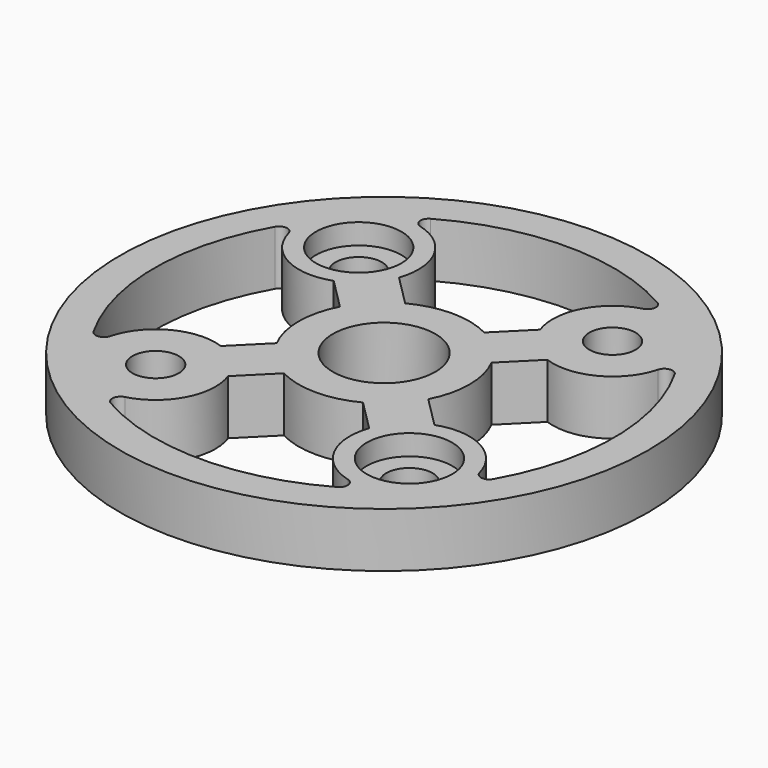
from build123d import *

# Parameters (mm, degrees)
F0_R            = 24.51608
F0_R_2          = 2.15265
F0_R_3          = 4.7625
F1_DEPTH        = 5.08
F3_DEPTH        = 5.08
F3_COPIES_COUNT = 4
F4_R            = 0.762
F6_R            = 3.96875
F7_DEPTH        = 1.905


# Not quite as in the source:
# - a pattern or mirror of a feature is missing from the dataset's text; its kind, count and spacing are read off the source's solid


with BuildPart() as f1:
    # F0 (on Top) → F1 (new body)
    with BuildSketch(Plane.XY):
        Circle(F0_R)
        with Locations((-11.7865906, -11.7865906)):
            Circle(F0_R_2, mode=Mode.SUBTRACT)
        with Locations((11.7865906, -11.7865906)):
            Circle(F0_R_2, mode=Mode.SUBTRACT)
        with Locations((-11.7865906, 11.7865906)):
            Circle(F0_R_2, mode=Mode.SUBTRACT)
        Circle(F0_R_3, mode=Mode.SUBTRACT)
        with Locations((11.7865906, 11.7865906)):
            Circle(F0_R_2, mode=Mode.SUBTRACT)
    extrude(amount=F1_DEPTH)

    # F2 (on face) → F3 (cut, through all)
    with BuildSketch(Plane.XY.offset(5.08)):
        with BuildLine():
            ThreePointArc((-12.5005198818, 17.2967828873), (-7.4612395718, 15.2741760893), (-6.553034663, 9.9206307084))
            Line((-6.553034663, 9.9206307084), (-3.6703384477, 7.0379344931))
            ThreePointArc((-3.6703384477, 7.0379344931), (0, 7.9375), (3.6703384477, 7.0379344931))
            Line((3.6703384477, 7.0379344931), (6.553034663, 9.9206307084))
            ThreePointArc((6.553034663, 9.9206307084), (7.4612395718, 15.2741760893), (12.5005198818, 17.2967828873))
            ThreePointArc((12.5005198818, 17.2967828873), (0, 21.34108), (-12.5005198818, 17.2967828873))
        make_face()
    f3 = extrude(amount=-F3_DEPTH, mode=Mode.SUBTRACT)

    # F3_copies: F3 ×4 about axis
    f3_copies_axis = Axis((0, 0, 0), (0, 0, 1))
    for i in range(1, F3_COPIES_COUNT):
        add(f3.rotate(f3_copies_axis, i * 360 / F3_COPIES_COUNT), mode=Mode.SUBTRACT)

    # F4
    f4_edges = [f1.edges().sort_by_distance(p)[0] for p in [
        (-12.50052, 17.296783, 2.54),
        (12.50052, 17.296783, 2.54),
        (-17.296783, -12.50052, 2.54),
        (-17.296783, 12.50052, 2.54),
        (12.50052, -17.296783, 2.54),
        (-12.50052, -17.296783, 2.54),
        (17.296783, 12.50052, 2.54),
        (17.296783, -12.50052, 2.54),
    ]]
    fillet(f4_edges, radius=F4_R)

    # F6 (on face) → F7 (cut, through all)
    with BuildSketch(Plane.XY.offset(5.08)):
        with Locations((11.7865906, -11.7865906)):
            Circle(F6_R)
        with Locations((-11.7865906, 11.7865906)):
            Circle(F6_R)
    extrude(amount=-F7_DEPTH, mode=Mode.SUBTRACT)


solid = f1.part
